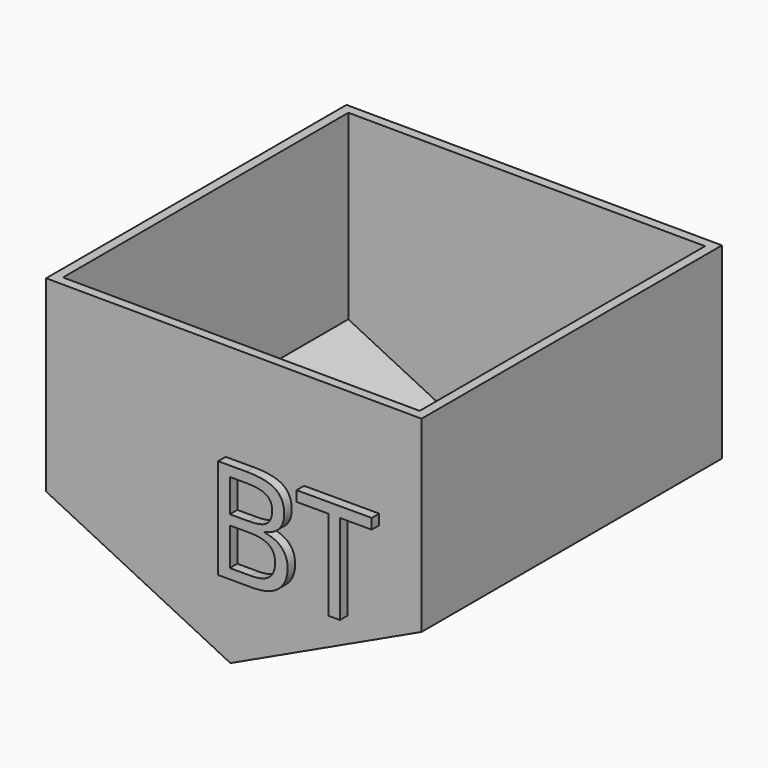
from build123d import *

# Parameters (mm, degrees)
F1_DEPTH     = 101.6
F2_T         = -2.54
F3_TEXT_SIZE = 37.9883994659
F4_DEPTH     = 2.54


# Not quite as in the source:
# - Text() gives the source's letters only with a copy of the font that has no kerning and outlines rounded to 1/6400 em; it was checked with that copy


with BuildPart() as f1:
    # F0 (on Front) → F1 (new body)
    with BuildSketch(Plane.XZ):
        Polygon((51.7188913369, 44.705352219), (-49.8802438378, 45.1245559349), (-49.8802438378, -5.6754440651), (0, -30.3395688534), (51.7188913369, -6.094647781), align=None)
    extrude(amount=F1_DEPTH)

    # F2
    f2_openings = [f1.faces().sort_by_distance(p)[0] for p in [
        (0.919324, -50.8, 44.914954),
    ]]
    offset(amount=F2_T, openings=f2_openings)

    # F3 (on face) → F4 (join)
    with BuildSketch(Plane.XZ.offset(101.6)):
        with Locations((-5.0249262713, -8.7416097522)):
            Text('BT', F3_TEXT_SIZE, font='Open Sans', text_align=(TextAlign.LEFT, TextAlign.BOTTOM))
    extrude(amount=F4_DEPTH)


solid = f1.part
